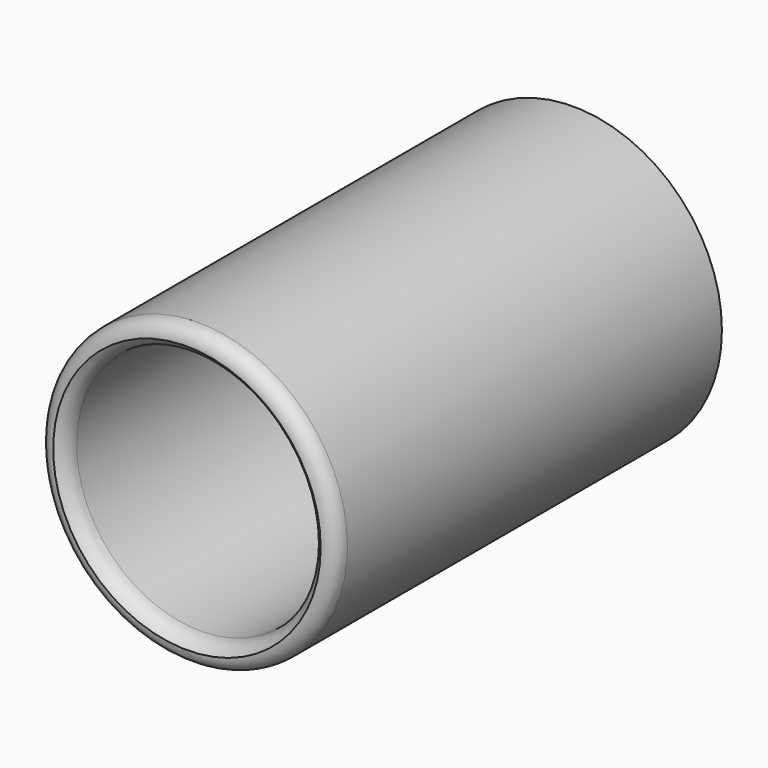
from build123d import *

# Parameters (mm, degrees)
F0_R     = 38.1
F0_R_2   = 31.75
F1_DEPTH = 123.825
F2_DEPTH = 9.525
F3_R     = 3.81
F5_DEPTH = 5.08
F6_R     = 2.53999


# Not quite as in the source:
# - a fillet or chamfer that OpenCascade refuses, or shapes differently, is made with other operations: its cross-section is extruded or revolved along the edge and cut away or added
# - a fillet or chamfer is up to 0.001 mm smaller than in the source, because OpenCascade refuses the exact size


with BuildPart() as f1:
    # F0 (on Front) → F1 (new body)
    with BuildSketch(Plane.XZ):
        Circle(F0_R)
        Circle(F0_R_2, mode=Mode.SUBTRACT)
    extrude(amount=F1_DEPTH)

    # F0 (on Front) → F2 (join)
    with BuildSketch(Plane.XZ):
        Circle(F0_R_2)
    extrude(amount=F2_DEPTH)

    # F3
    f3_edges = [f1.edges().sort_by_distance(p)[0] for p in [
        (-38.1, -123.825, 0),
    ]]
    fillet(f3_edges, radius=F3_R)

    # F4: fillet of radius 5.08 on 1 edges, made by hand

    # F4_s1 → F4_t2 (revolve, cut)
    with BuildSketch(Plane.XY):
        with BuildLine():
            ThreePointArc((34.289799962, -123.8253463882), (32.4302345225, -121.9654748362), (31.7496, -119.4250334454))
            Line((31.7496, -119.4250334454), (31.2414634315, -119.4250334454))
            ThreePointArc((31.2414634315, -119.4250334454), (31.2418634315, -121.6250167227), (31.2418634315, -123.825))
            Line((31.2418634315, -123.825), (31.75, -124.3331365685))
            ThreePointArc((31.75, -124.3331365685), (33.019899981, -124.3331365685), (34.0356833896, -124.2653776825))
            Line((34.0356833896, -124.2653776825), (34.289799962, -123.8253463882))
        make_face()
    revolve(axis=Axis((0, -123.825, 0), (0, -1, 0)), mode=Mode.SUBTRACT)

    # F0 (on Front) → F5 (cut)
    with BuildSketch(Plane.XZ):
        Circle(F0_R_2)
    extrude(amount=F5_DEPTH, mode=Mode.SUBTRACT)

    # F6 (radius 2.54 in the source; OpenCascade refuses exactly that, so slightly less here)
    f6_edges = [f1.edges().sort_by_distance(p)[0] for p in [
        (-31.75, -5.08, 0),
        (-31.75, 0, 0),
    ]]
    fillet(f6_edges, radius=F6_R)


solid = f1.part
